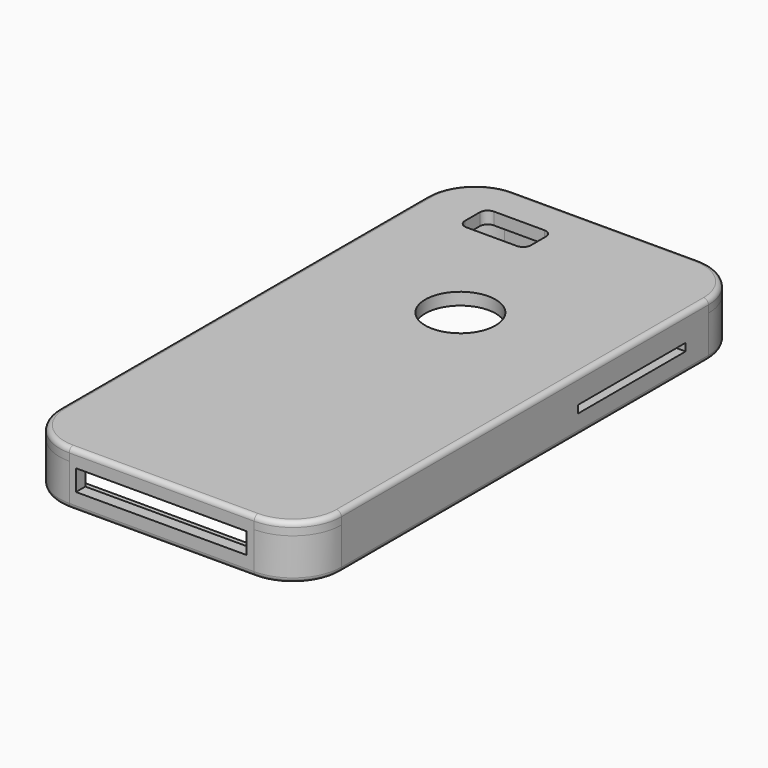
from build123d import *

# Parameters (mm, degrees)
F0_R       = 9.1313
F1_DEPTH   = 7.7089
F2_W       = 9.779
F2_H       = 1.9812
F3_DEPTH   = 9.144
F4_W       = 44.2985175177
F4_H       = 5.4359880742
F5_DEPTH   = 17.018
F6_W       = 34.925
F6_H       = 1.9812
F7_DEPTH   = 68.834
F8_DEPTH   = 7.7089
F9_DEPTH   = 32.004
F10_DEPTH  = 3.175
F1_FACE2_R = 9.1313
F11_DEPTH  = 3.175
F13_R      = 1.27


with BuildPart() as f1:
    # F0 (on Top) → F1 (new body)
    with BuildSketch(Plane.XY):
        with BuildLine():
            Line((11.6091579572, 58.7859712541), (-36.4349420428, 58.7859712541))
            ThreePointArc((-36.4349420428, 58.7859712541), (-43.1701341336, 55.9961633449), (-45.9599420428, 49.2609712541))
            Line((-45.9599420428, 49.2609712541), (-45.9599420428, -69.9285287459))
            ThreePointArc((-45.9599420428, -69.9285287459), (-43.1701341336, -76.6637208367), (-36.4349420428, -79.4535287459))
            Line((-36.4349420428, -79.4535287459), (11.6091579572, -79.4535287459))
            ThreePointArc((11.6091579572, -79.4535287459), (18.344350048, -76.6637208367), (21.1341579572, -69.9285287459))
            Line((21.1341579572, -69.9285287459), (21.1341579572, 29.7156712541))
            Line((21.1341579572, 29.7156712541), (21.1341579572, 49.2609712541))
            ThreePointArc((21.1341579572, 49.2609712541), (18.344350048, 55.9961633449), (11.6091579572, 58.7859712541))
        make_face()
        with BuildLine():
            ThreePointArc((-42.9119420428, 49.2609712541), (-41.0148726646, 53.8409018759), (-36.4349420428, 55.7379712541))
            Line((-36.4349420428, 55.7379712541), (11.6091579572, 55.7379712541))
            ThreePointArc((11.6091579572, 55.7379712541), (16.1890885789, 53.8409018759), (18.0861579572, 49.2609712541))
            Line((18.0861579572, 49.2609712541), (18.0861579572, -69.9285287459))
            ThreePointArc((18.0861579572, -69.9285287459), (16.1890885789, -74.5084593676), (11.6091579572, -76.4055287459))
            Line((11.6091579572, -76.4055287459), (-36.4349420428, -76.4055287459))
            ThreePointArc((-36.4349420428, -76.4055287459), (-41.0148726646, -74.5084593676), (-42.9119420428, -69.9285287459))
            Line((-42.9119420428, -69.9285287459), (-42.9119420428, 49.2609712541))
        make_face(mode=Mode.SUBTRACT)
        with BuildLine():
            Line((11.6091579572, 55.7379712541), (-36.4349420428, 55.7379712541))
            ThreePointArc((-36.4349420428, 55.7379712541), (-41.0148726646, 53.8409018759), (-42.9119420428, 49.2609712541))
            Line((-42.9119420428, 49.2609712541), (-42.9119420428, -69.9285287459))
            ThreePointArc((-42.9119420428, -69.9285287459), (-41.0148726646, -74.5084593676), (-36.4349420428, -76.4055287459))
            Line((-36.4349420428, -76.4055287459), (11.6091579572, -76.4055287459))
            ThreePointArc((11.6091579572, -76.4055287459), (16.1890885789, -74.5084593676), (18.0861579572, -69.9285287459))
            Line((18.0861579572, -69.9285287459), (18.0861579572, 49.2609712541))
            ThreePointArc((18.0861579572, 49.2609712541), (16.1890885789, 53.8409018759), (11.6091579572, 55.7379712541))
        make_face()
        with BuildLine():
            Line((-35.9269420428, 45.3239712541), (-35.9269420428, 50.1753712541))
            ThreePointArc((-35.9269420428, 50.1753712541), (-35.3317830222, 51.6122122335), (-33.8949420428, 52.2073712541))
            Line((-33.8949420428, 52.2073712541), (-20.8139420428, 52.2073712541))
            ThreePointArc((-20.8139420428, 52.2073712541), (-19.3771010635, 51.6122122335), (-18.7819420428, 50.1753712541))
            Line((-18.7819420428, 50.1753712541), (-18.7819420428, 45.3239712541))
            ThreePointArc((-18.7819420428, 45.3239712541), (-19.3771010635, 43.8871302747), (-20.8139420428, 43.2919712541))
            Line((-20.8139420428, 43.2919712541), (-33.8949420428, 43.2919712541))
            ThreePointArc((-33.8949420428, 43.2919712541), (-35.3317830222, 43.8871302747), (-35.9269420428, 45.3239712541))
        make_face(mode=Mode.SUBTRACT)
        with Locations((-11.4921420428, 13.3246481419)):
            Circle(F0_R, mode=Mode.SUBTRACT)
    extrude(amount=F1_DEPTH)

    # F4 (on face) → F5 (join)
    with BuildSketch(Plane.XZ.offset(79.4535287459)):
        with Locations((-12.5446827151, 3.9651609259)):
            Rectangle(F4_W, F4_H)
    extrude(amount=F5_DEPTH)

    # F0 (on Top) → F9 (join)
    with BuildSketch(Plane.XY):
        with BuildLine():
            Line((11.6091579572, 55.7379712541), (-36.4349420428, 55.7379712541))
            ThreePointArc((-36.4349420428, 55.7379712541), (-41.0148726646, 53.8409018759), (-42.9119420428, 49.2609712541))
            Line((-42.9119420428, 49.2609712541), (-42.9119420428, -69.9285287459))
            ThreePointArc((-42.9119420428, -69.9285287459), (-41.0148726646, -74.5084593676), (-36.4349420428, -76.4055287459))
            Line((-36.4349420428, -76.4055287459), (11.6091579572, -76.4055287459))
            ThreePointArc((11.6091579572, -76.4055287459), (16.1890885789, -74.5084593676), (18.0861579572, -69.9285287459))
            Line((18.0861579572, -69.9285287459), (18.0861579572, 49.2609712541))
            ThreePointArc((18.0861579572, 49.2609712541), (16.1890885789, 53.8409018759), (11.6091579572, 55.7379712541))
        make_face()
        with BuildLine():
            Line((-35.9269420428, 45.3239712541), (-35.9269420428, 50.1753712541))
            ThreePointArc((-35.9269420428, 50.1753712541), (-35.3317830222, 51.6122122335), (-33.8949420428, 52.2073712541))
            Line((-33.8949420428, 52.2073712541), (-20.8139420428, 52.2073712541))
            ThreePointArc((-20.8139420428, 52.2073712541), (-19.3771010635, 51.6122122335), (-18.7819420428, 50.1753712541))
            Line((-18.7819420428, 50.1753712541), (-18.7819420428, 45.3239712541))
            ThreePointArc((-18.7819420428, 45.3239712541), (-19.3771010635, 43.8871302747), (-20.8139420428, 43.2919712541))
            Line((-20.8139420428, 43.2919712541), (-33.8949420428, 43.2919712541))
            ThreePointArc((-33.8949420428, 43.2919712541), (-35.3317830222, 43.8871302747), (-35.9269420428, 45.3239712541))
        make_face(mode=Mode.SUBTRACT)
        with Locations((-11.4921420428, 13.3246481419)):
            Circle(F0_R, mode=Mode.SUBTRACT)
    extrude(amount=-F9_DEPTH)


with BuildPart() as f3:
    # F2 (on face) → F3 (new body)
    with BuildSketch(Plane(origin=(-45.9599420428, 0, 0), x_dir=(0, -1, 0), z_dir=(-1, 0, 0))):
        with Locations((-25.3214712541, 2.974975)):
            Rectangle(F2_W, F2_H)
    extrude(amount=F3_DEPTH)


with BuildPart() as f7:
    # F6 (on Right) → F7 (new body)
    with BuildSketch(Plane.YZ):
        with Locations((24.3882495925, 2.974975)):
            Rectangle(F6_W, F6_H)
    extrude(amount=F7_DEPTH)


with BuildPart() as f8:
    # F0 (on Top) → F8 (new body, through all)
    with BuildSketch(Plane.XY):
        with BuildLine():
            Line((24.1821579572, -69.9285287459), (24.1821579572, 49.2609712541))
            ThreePointArc((24.1821579572, 49.2609712541), (20.499611517, 58.151424814), (11.6091579572, 61.8339712541))
            Line((11.6091579572, 61.8339712541), (-36.4349420428, 61.8339712541))
            ThreePointArc((-36.4349420428, 61.8339712541), (-45.3253956027, 58.151424814), (-49.0079420428, 49.2609712541))
            Line((-49.0079420428, 49.2609712541), (-49.0079420428, -69.9285287459))
            ThreePointArc((-49.0079420428, -69.9285287459), (-45.3253956027, -78.8189823057), (-36.4349420428, -82.5015287459))
            Line((-36.4349420428, -82.5015287459), (11.6091579572, -82.5015287459))
            ThreePointArc((11.6091579572, -82.5015287459), (20.499611517, -78.8189823057), (24.1821579572, -69.9285287459))
        make_face()
        with BuildLine():
            ThreePointArc((-45.9599420428, 49.2609712541), (-43.1701341336, 55.9961633449), (-36.4349420428, 58.7859712541))
            Line((-36.4349420428, 58.7859712541), (11.6091579572, 58.7859712541))
            ThreePointArc((11.6091579572, 58.7859712541), (18.344350048, 55.9961633449), (21.1341579572, 49.2609712541))
            Line((21.1341579572, 49.2609712541), (21.1341579572, 29.7156712541))
            Line((21.1341579572, 29.7156712541), (21.1341579572, -69.9285287459))
            ThreePointArc((21.1341579572, -69.9285287459), (18.344350048, -76.6637208367), (11.6091579572, -79.4535287459))
            Line((11.6091579572, -79.4535287459), (-36.4349420428, -79.4535287459))
            ThreePointArc((-36.4349420428, -79.4535287459), (-43.1701341336, -76.6637208367), (-45.9599420428, -69.9285287459))
            Line((-45.9599420428, -69.9285287459), (-45.9599420428, 49.2609712541))
        make_face(mode=Mode.SUBTRACT)
    extrude(amount=F8_DEPTH)

    # F0 (on Top) → F10 (join)
    with BuildSketch(Plane.XY):
        with BuildLine():
            Line((24.1821579572, -69.9285287459), (24.1821579572, 49.2609712541))
            ThreePointArc((24.1821579572, 49.2609712541), (20.499611517, 58.151424814), (11.6091579572, 61.8339712541))
            Line((11.6091579572, 61.8339712541), (-36.4349420428, 61.8339712541))
            ThreePointArc((-36.4349420428, 61.8339712541), (-45.3253956027, 58.151424814), (-49.0079420428, 49.2609712541))
            Line((-49.0079420428, 49.2609712541), (-49.0079420428, -69.9285287459))
            ThreePointArc((-49.0079420428, -69.9285287459), (-45.3253956027, -78.8189823057), (-36.4349420428, -82.5015287459))
            Line((-36.4349420428, -82.5015287459), (11.6091579572, -82.5015287459))
            ThreePointArc((11.6091579572, -82.5015287459), (20.499611517, -78.8189823057), (24.1821579572, -69.9285287459))
        make_face()
        with BuildLine():
            ThreePointArc((-45.9599420428, 49.2609712541), (-43.1701341336, 55.9961633449), (-36.4349420428, 58.7859712541))
            Line((-36.4349420428, 58.7859712541), (11.6091579572, 58.7859712541))
            ThreePointArc((11.6091579572, 58.7859712541), (18.344350048, 55.9961633449), (21.1341579572, 49.2609712541))
            Line((21.1341579572, 49.2609712541), (21.1341579572, 29.7156712541))
            Line((21.1341579572, 29.7156712541), (21.1341579572, -69.9285287459))
            ThreePointArc((21.1341579572, -69.9285287459), (18.344350048, -76.6637208367), (11.6091579572, -79.4535287459))
            Line((11.6091579572, -79.4535287459), (-36.4349420428, -79.4535287459))
            ThreePointArc((-36.4349420428, -79.4535287459), (-43.1701341336, -76.6637208367), (-45.9599420428, -69.9285287459))
            Line((-45.9599420428, -69.9285287459), (-45.9599420428, 49.2609712541))
        make_face(mode=Mode.SUBTRACT)
        with BuildLine():
            Line((11.6091579572, 58.7859712541), (-36.4349420428, 58.7859712541))
            ThreePointArc((-36.4349420428, 58.7859712541), (-43.1701341336, 55.9961633449), (-45.9599420428, 49.2609712541))
            Line((-45.9599420428, 49.2609712541), (-45.9599420428, -69.9285287459))
            ThreePointArc((-45.9599420428, -69.9285287459), (-43.1701341336, -76.6637208367), (-36.4349420428, -79.4535287459))
            Line((-36.4349420428, -79.4535287459), (11.6091579572, -79.4535287459))
            ThreePointArc((11.6091579572, -79.4535287459), (18.344350048, -76.6637208367), (21.1341579572, -69.9285287459))
            Line((21.1341579572, -69.9285287459), (21.1341579572, 29.7156712541))
            Line((21.1341579572, 29.7156712541), (21.1341579572, 49.2609712541))
            ThreePointArc((21.1341579572, 49.2609712541), (18.344350048, 55.9961633449), (11.6091579572, 58.7859712541))
        make_face()
        with BuildLine():
            ThreePointArc((-42.9119420428, 49.2609712541), (-41.0148726646, 53.8409018759), (-36.4349420428, 55.7379712541))
            Line((-36.4349420428, 55.7379712541), (11.6091579572, 55.7379712541))
            ThreePointArc((11.6091579572, 55.7379712541), (16.1890885789, 53.8409018759), (18.0861579572, 49.2609712541))
            Line((18.0861579572, 49.2609712541), (18.0861579572, -69.9285287459))
            ThreePointArc((18.0861579572, -69.9285287459), (16.1890885789, -74.5084593676), (11.6091579572, -76.4055287459))
            Line((11.6091579572, -76.4055287459), (-36.4349420428, -76.4055287459))
            ThreePointArc((-36.4349420428, -76.4055287459), (-41.0148726646, -74.5084593676), (-42.9119420428, -69.9285287459))
            Line((-42.9119420428, -69.9285287459), (-42.9119420428, 49.2609712541))
        make_face(mode=Mode.SUBTRACT)
    extrude(amount=-F10_DEPTH)

    # F1_face2 (on face) + F8_face (on face) → F11 (join)
    with BuildSketch(Plane(origin=(-12.1864232074, -12.0262288376, 7.7089), x_dir=(1, 0, 0), z_dir=(0, 0, 1))):
        with BuildLine():
            Line((23.7955811646, 70.8122000917), (-24.2485188354, 70.8122000917))
            ThreePointArc((-24.2485188354, 70.8122000917), (-30.9837109262, 68.0223921825), (-33.7735188354, 61.2872000917))
            Line((-33.7735188354, 61.2872000917), (-33.7735188354, -57.9022999083))
            ThreePointArc((-33.7735188354, -57.9022999083), (-30.9837109262, -64.6374919991), (-24.2485188354, -67.4272999083))
            Line((-24.2485188354, -67.4272999083), (23.7955811646, -67.4272999083))
            ThreePointArc((23.7955811646, -67.4272999083), (30.5307732554, -64.6374919991), (33.3205811646, -57.9022999083))
            Line((33.3205811646, -57.9022999083), (33.3205811646, 61.2872000917))
            ThreePointArc((33.3205811646, 61.2872000917), (30.5307732554, 68.0223921825), (23.7955811646, 70.8122000917))
        make_face()
        with BuildLine():
            Line((-8.6275188354, 55.3182000917), (-21.7085188354, 55.3182000917))
            ThreePointArc((-21.7085188354, 55.3182000917), (-23.1453598148, 55.9133591123), (-23.7405188354, 57.3502000917))
            Line((-23.7405188354, 57.3502000917), (-23.7405188354, 62.2016000917))
            ThreePointArc((-23.7405188354, 62.2016000917), (-23.1453598148, 63.6384410711), (-21.7085188354, 64.2336000917))
            Line((-21.7085188354, 64.2336000917), (-8.6275188354, 64.2336000917))
            ThreePointArc((-8.6275188354, 64.2336000917), (-7.1906778561, 63.6384410711), (-6.5955188354, 62.2016000917))
            Line((-6.5955188354, 62.2016000917), (-6.5955188354, 57.3502000917))
            ThreePointArc((-6.5955188354, 57.3502000917), (-7.1906778561, 55.9133591123), (-8.6275188354, 55.3182000917))
        make_face(mode=Mode.SUBTRACT)
        with Locations((0.6942811646, 25.3508769795)):
            Circle(F1_FACE2_R, mode=Mode.SUBTRACT)
    with BuildSketch(Plane(origin=(-12.4128920428, -10.3337787459, 7.7089), x_dir=(1, 0, 0), z_dir=(0, 0, 1))):
        with BuildLine():
            Line((36.59505, -59.59475), (36.59505, 59.59475))
            ThreePointArc((36.59505, 59.59475), (32.9125035599, 68.4852035599), (24.02205, 72.16775))
            Line((24.02205, 72.16775), (-24.02205, 72.16775))
            ThreePointArc((-24.02205, 72.16775), (-32.9125035599, 68.4852035599), (-36.59505, 59.59475))
            Line((-36.59505, 59.59475), (-36.59505, -59.59475))
            ThreePointArc((-36.59505, -59.59475), (-32.9125035599, -68.4852035599), (-24.02205, -72.16775))
            Line((-24.02205, -72.16775), (24.02205, -72.16775))
            ThreePointArc((24.02205, -72.16775), (32.9125035599, -68.4852035599), (36.59505, -59.59475))
        make_face()
        with BuildLine():
            ThreePointArc((-33.54705, 59.59475), (-30.7572420908, 66.3299420908), (-24.02205, 69.11975))
            Line((-24.02205, 69.11975), (24.02205, 69.11975))
            ThreePointArc((24.02205, 69.11975), (30.7572420908, 66.3299420908), (33.54705, 59.59475))
            Line((33.54705, 59.59475), (33.54705, -59.59475))
            ThreePointArc((33.54705, -59.59475), (30.7572420908, -66.3299420908), (24.02205, -69.11975))
            Line((24.02205, -69.11975), (-24.02205, -69.11975))
            ThreePointArc((-24.02205, -69.11975), (-30.7572420908, -66.3299420908), (-33.54705, -59.59475))
            Line((-33.54705, -59.59475), (-33.54705, 59.59475))
        make_face(mode=Mode.SUBTRACT)
    extrude(amount=F11_DEPTH)

    # F12: cut F3, F7, F1
    add(f3.part, mode=Mode.SUBTRACT)
    add(f7.part, mode=Mode.SUBTRACT)
    add(f1.part, mode=Mode.SUBTRACT)

    # F13
    f13_edges = [f8.edges().sort_by_distance(p)[0] for p in [
        (-49.007942, -10.333779, -3.175),
        (-45.325396, -78.818982, -3.175),
        (-49.007942, -10.333779, 10.8839),
        (-12.412892, 55.737971, -3.175),
        (24.182158, -10.333779, 10.8839),
        (24.182158, -10.333779, -3.175),
        (20.499612, -78.818982, 10.8839),
        (20.499612, -78.818982, -3.175),
        (20.499612, 58.151425, 10.8839),
        (-12.412892, 61.833971, 10.8839),
        (-45.325396, 58.151425, 10.8839),
        (-45.325396, -78.818982, 10.8839),
        (-12.412892, -82.501529, 10.8839),
        (-41.014873, 53.840902, -3.175),
        (16.189089, 53.840902, -3.175),
        (18.086158, -10.333779, -3.175),
        (16.189089, -74.508459, -3.175),
        (-12.412892, -76.405529, -3.175),
        (-41.014873, -74.508459, -3.175),
        (-42.911942, -10.333779, -3.175),
        (20.499612, 58.151425, -3.175),
        (-12.412892, 61.833971, -3.175),
        (-45.325396, 58.151425, -3.175),
        (-12.412892, -82.501529, -3.175),
    ]]
    fillet(f13_edges, radius=F13_R)


solid = f8.part
